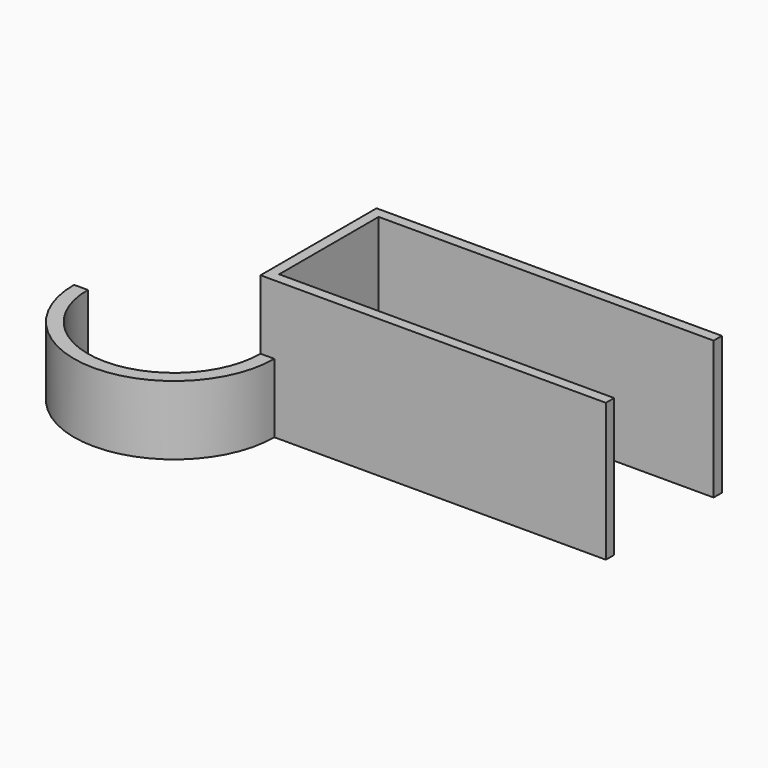
from build123d import *

# Parameters (mm, degrees)
F1_DEPTH = 20
F2_DEPTH = 10


# Not quite as in the source:
# - a feature names something its author has since deleted; it is built from what else it names


with BuildPart() as f1:
    # F0 (on Top) → F1 (new body)
    with BuildSketch(Plane.XY):
        Polygon((-50, 21), (-50, 0), (-48, 0), (0, 0), (0, 1.5), (-48.5, 1.5), (-48.5, 19.5), (0, 19.5), (0, 21), align=None)
    extrude(amount=F1_DEPTH)

    # F0 (on Top) → F2 (join)
    with BuildSketch(Plane.XY):
        with BuildLine():
            ThreePointArc((-50, 0), (-62.5, -12.5), (-75, 0))
            Line((-75, 0), (-77, 0))
            ThreePointArc((-77, 0), (-62.5, -14.5), (-48, 0))
            Line((-48, 0), (-50, 0))
        make_face()
    extrude(amount=F2_DEPTH)


solid = f1.part
